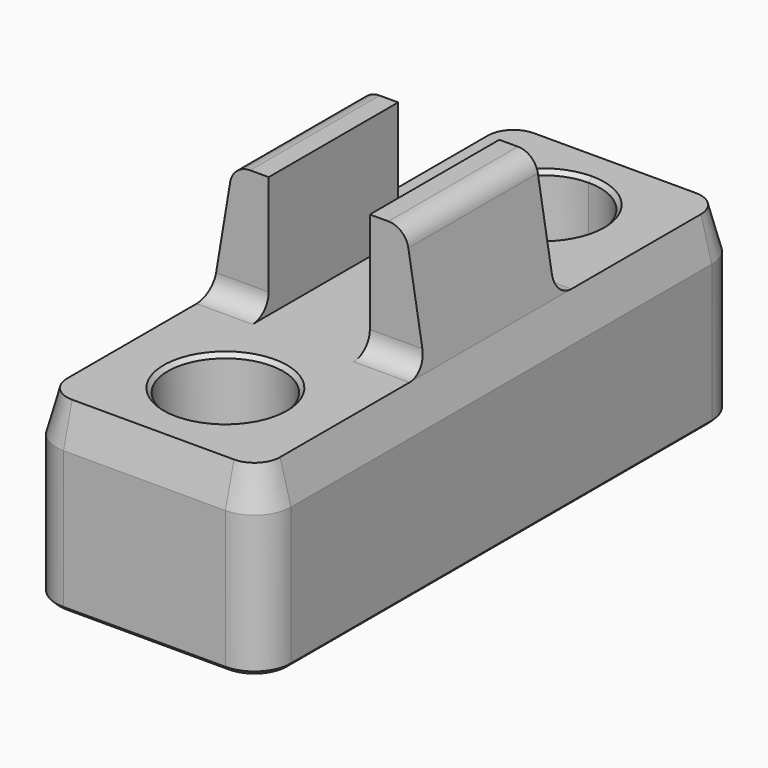
from build123d import *

# Parameters (mm, degrees)
F1_DEPTH      = 9
F3_DEPTH      = 25
F4_DEPTH      = 3.2
F5_SIZE       = 0.2
F6_SIZE2      = 0.5358983849
F6_SIZE       = 2
F7_W          = 2.7641016151
F7_H          = 6
F8_DEPTH      = 6
F9_T4_DEPTH   = 37.1842967295
F9_T9_DEPTH   = 37.1842967295
F10_DEPTH     = 1
F11_DEPTH     = 1
F12_T4_DEPTH  = 5.2641016151
F12_T10_DEPTH = 5.2641016151
F12_T16_DEPTH = 5.2641016151
F12_T22_DEPTH = 5.2641016151
F12_T28_DEPTH = 5.2641016151
F12_T34_DEPTH = 5.2641016151
F12_T40_DEPTH = 5.2641016151
F12_T46_DEPTH = 5.2641016151
F12_T49_DEPTH = 12.2356354419


# Not quite as in the source:
# - a fillet or chamfer that OpenCascade refuses, or shapes differently, is made with other operations: its cross-section is extruded or revolved along the edge and cut away or added


with BuildPart() as f1:
    # F0 (on Top) → F1 (new body)
    with BuildSketch(Plane.XY):
        with BuildLine():
            Line((-34.4771644294, 42.6813552976), (-34.4771644294, 68.6813552976))
            ThreePointArc((-34.4771644294, 68.6813552976), (-35.0043722233, 69.9541475037), (-36.2771644294, 70.4813552976))
            Line((-36.2771644294, 70.4813552976), (-44.2771644294, 70.4813552976))
            ThreePointArc((-44.2771644294, 70.4813552976), (-45.5499566356, 69.9541475037), (-46.0771644294, 68.6813552976))
            Line((-46.0771644294, 68.6813552976), (-46.0771644294, 42.6813552976))
            ThreePointArc((-46.0771644294, 42.6813552976), (-45.5499566356, 41.4085630914), (-44.2771644294, 40.8813552976))
            Line((-44.2771644294, 40.8813552976), (-36.2771644294, 40.8813552976))
            ThreePointArc((-36.2771644294, 40.8813552976), (-35.0043722233, 41.4085630914), (-34.4771644294, 42.6813552976))
        make_face()
    extrude(amount=F1_DEPTH)

    # F2 (on face) → F3 (cut)
    with BuildSketch(Plane.XY.offset(9)):
        with BuildLine():
            ThreePointArc((-38.7771644294, 65.4813552976), (-39.2165042576, 66.5420154693), (-40.2771644294, 66.9813552976))
            ThreePointArc((-40.2771644294, 66.9813552976), (-41.3378246012, 64.4206951258), (-38.7771644294, 65.4813552976))
        make_face()
        with BuildLine():
            ThreePointArc((-38.7771644294, 45.8813552976), (-41.3378246012, 46.9420154693), (-40.2771644294, 44.3813552976))
            ThreePointArc((-40.2771644294, 44.3813552976), (-39.2165042576, 44.8206951258), (-38.7771644294, 45.8813552976))
        make_face()
    extrude(amount=-F3_DEPTH, mode=Mode.SUBTRACT)

    # F2 (on face) → F4 (cut)
    with BuildSketch(Plane.XY.offset(9)):
        with BuildLine():
            ThreePointArc((-37.4271644294, 65.4813552976), (-38.261910103, 67.4966096239), (-40.2771644294, 68.3313552976))
            ThreePointArc((-40.2771644294, 68.3313552976), (-42.2924187558, 63.4661009712), (-37.4271644294, 65.4813552976))
        make_face()
        with BuildLine():
            ThreePointArc((-38.7771644294, 65.4813552976), (-41.3378246012, 64.4206951258), (-40.2771644294, 66.9813552976))
            ThreePointArc((-40.2771644294, 66.9813552976), (-39.2165042576, 66.5420154693), (-38.7771644294, 65.4813552976))
        make_face(mode=Mode.SUBTRACT)
        with BuildLine():
            ThreePointArc((-37.4271644294, 45.8813552976), (-42.2924187558, 47.8966096239), (-40.2771644294, 43.0313552976))
            ThreePointArc((-40.2771644294, 43.0313552976), (-38.261910103, 43.8661009712), (-37.4271644294, 45.8813552976))
        make_face()
        with BuildLine():
            ThreePointArc((-38.7771644294, 45.8813552976), (-39.2165042576, 44.8206951258), (-40.2771644294, 44.3813552976))
            ThreePointArc((-40.2771644294, 44.3813552976), (-41.3378246012, 46.9420154693), (-38.7771644294, 45.8813552976))
        make_face(mode=Mode.SUBTRACT)
    extrude(amount=-F4_DEPTH, mode=Mode.SUBTRACT)

    # F5
    f5_edges = [f1.edges().sort_by_distance(p)[0] for p in [
        (-40.277164, 63.981355, 5.8),
        (-40.277164, 47.381355, 5.8),
        (-34.477164, 55.681355, 0),
        (-35.004372, 41.408563, 0),
        (-35.004372, 69.954148, 0),
        (-40.277164, 40.881355, 0),
        (-40.277164, 70.481355, 0),
        (-45.549957, 41.408563, 0),
        (-45.549957, 69.954148, 0),
        (-46.077164, 55.681355, 0),
        (-40.277164, 47.381355, 0),
        (-40.277164, 63.981355, 0),
        (-40.277164, 62.631355, 9),
        (-40.277164, 48.731355, 9),
    ]]
    chamfer(f5_edges, length=F5_SIZE)

    # F6
    f6_edges = [f1.edges().sort_by_distance(p)[0] for p in [
        (-34.477164, 55.681355, 9),
    ]]
    f6_side = f1.faces().sort_by_distance((-34.477164, 55.681355, 4.6))[0]
    chamfer(f6_edges, length=F6_SIZE, length2=F6_SIZE2, reference=f6_side)

    # F7 (on face) → F8 (join)
    with BuildSketch(Plane.XY.offset(9)):
        with Locations((-36.3951136219, 55.6813552976)):
            Rectangle(F7_W, F7_H)
        with Locations((-44.159215237, 55.6813552976)):
            Rectangle(F7_W, F7_H)
    extrude(amount=F8_DEPTH)

    # F9: chamfer of 1 x 6 on 2 edges, made by hand


with BuildPart() as f9_tool2:
    # F9_s3 → F9_t4 (new body)
    with BuildSketch(Plane.XZ.offset(-37.0892069328)):
        Polygon((-35.0130628143, 9), (-36.0130628143, 15), (-35.0130628143, 15), align=None)
    extrude(amount=-F9_T4_DEPTH)

    split(bisect_by=Plane(origin=(-30.4176323379, 0, -8.1503800206), x_dir=(0, 1, 0), z_dir=(0.9659258263, 0, 0.2588190451)), keep=Keep.TOP)


with BuildPart() as f1_1:
    add(f1.part)

    # F9_t1: cut F9_tool2
    add(f9_tool2.part, mode=Mode.SUBTRACT)


with BuildPart() as f9_tool7:
    # F9_s8 → F9_t9 (new body)
    with BuildSketch(Plane.XZ.offset(-74.2735036623)):
        Polygon((-45.5412660446, 9), (-44.5412660446, 15), (-45.5412660446, 15), align=None)
    extrude(amount=F9_T9_DEPTH)

    split(bisect_by=Plane(origin=(-44.7405796798, 0, 11.9882021941), x_dir=(0, 1, 0), z_dir=(-0.9659258263, 0, 0.2588190451)), keep=Keep.TOP)


with BuildPart() as f1_2:
    add(f1_1.part)

    # F9_t6: cut F9_tool7
    add(f9_tool7.part, mode=Mode.SUBTRACT)

    # F10 (add): faces of the model
    f10_faces = [f1_2.faces().sort_by_distance(p)[0] for p in [
        (-36.6267104431, 58.6813552976, 11.7791618553),
        (-43.9276184157, 58.6813552976, 11.7791618553),
    ]]
    extrude(f10_faces, amount=F10_DEPTH)

    # F11 (add): faces of the model
    f11_faces = [f1_2.faces().sort_by_distance(p)[0] for p in [
        (-43.9276184157, 52.6813552976, 11.7791618553),
        (-36.6267104431, 52.6813552976, 11.7791618553),
    ]]
    extrude(f11_faces, amount=F11_DEPTH)

    # F12: fillet of radius 1 on 6 edges, made by hand


with BuildPart() as f12_tool2:
    # F12_s3 → F12_t4 (new body)
    with BuildSketch(Plane.YZ.offset(-37.7771644294)):
        with BuildLine():
            ThreePointArc((50.6813552976, 9), (51.3884620788, 9.2928932188), (51.6813552976, 10))
            Line((51.6813552976, 10), (51.6813552976, 9))
            Line((51.6813552976, 9), (50.6813552976, 9))
        make_face()
    extrude(amount=F12_T4_DEPTH)

    split(bisect_by=Plane(origin=(-30.4176323379, 0, -8.1503800206), x_dir=(0, 1, 0), z_dir=(-0.9659258263, 0, -0.2588190451)), keep=Keep.TOP)

    split(bisect_by=Plane(origin=(-32.6073043599, 0, -5.4345507266), x_dir=(0, 1, 0), z_dir=(-0.9863939238, 0, -0.1643989873)), keep=Keep.TOP)


with BuildPart() as f1_3:
    add(f1_2.part)

    # F12_t1: union F12_tool2
    add(f12_tool2.part)


with BuildPart() as f12_tool8:
    # F12_s9 → F12_t10 (new body)
    with BuildSketch(Plane.YZ.offset(-37.7771644294)):
        with BuildLine():
            ThreePointArc((50.6813552976, 9), (51.3884620788, 9.2928932188), (51.6813552976, 10))
            Line((51.6813552976, 10), (51.6813552976, 9))
            Line((51.6813552976, 9), (50.6813552976, 9))
        make_face()
    extrude(amount=F12_T10_DEPTH)

    split(bisect_by=Plane(origin=(-30.4176323379, 0, -8.1503800206), x_dir=(0, 1, 0), z_dir=(0.9659258263, 0, 0.2588190451)), keep=Keep.TOP)

    split(bisect_by=Plane(origin=(-32.6073043599, 0, -5.4345507266), x_dir=(0, 1, 0), z_dir=(-0.9863939238, 0, -0.1643989873)), keep=Keep.TOP)


with BuildPart() as f1_4:
    add(f1_3.part)

    # F12_t7: union F12_tool8
    add(f12_tool8.part)


with BuildPart() as f12_tool14:
    # F12_s15 → F12_t16 (new body)
    with BuildSketch(Plane.YZ.offset(-48.0412660446)):
        with BuildLine():
            ThreePointArc((50.6813552976, 9), (51.3884620788, 9.2928932188), (51.6813552976, 10))
            Line((51.6813552976, 10), (51.6813552976, 9))
            Line((51.6813552976, 9), (50.6813552976, 9))
        make_face()
    extrude(amount=F12_T16_DEPTH)

    split(bisect_by=Plane(origin=(-44.7405796798, 0, 11.9882021941), x_dir=(0, 1, 0), z_dir=(-0.9659258263, 0, 0.2588190451)), keep=Keep.TOP)

    split(bisect_by=Plane(origin=(-45.7698804758, 0, 7.6283134126), x_dir=(0, 1, 0), z_dir=(0.9863939238, 0, -0.1643989873)), keep=Keep.TOP)


with BuildPart() as f1_5:
    add(f1_4.part)

    # F12_t13: union F12_tool14
    add(f12_tool14.part)


with BuildPart() as f12_tool20:
    # F12_s21 → F12_t22 (new body)
    with BuildSketch(Plane.YZ.offset(-48.0412660446)):
        with BuildLine():
            ThreePointArc((50.6813552976, 9), (51.3884620788, 9.2928932188), (51.6813552976, 10))
            Line((51.6813552976, 10), (51.6813552976, 9))
            Line((51.6813552976, 9), (50.6813552976, 9))
        make_face()
    extrude(amount=F12_T22_DEPTH)

    split(bisect_by=Plane(origin=(-44.7405796798, 0, 11.9882021941), x_dir=(0, 1, 0), z_dir=(0.9659258263, 0, -0.2588190451)), keep=Keep.TOP)

    split(bisect_by=Plane(origin=(-45.7698804758, 0, 7.6283134126), x_dir=(0, 1, 0), z_dir=(0.9863939238, 0, -0.1643989873)), keep=Keep.TOP)


with BuildPart() as f1_6:
    add(f1_5.part)

    # F12_t19: union F12_tool20
    add(f12_tool20.part)


with BuildPart() as f12_tool26:
    # F12_s27 → F12_t28 (new body)
    with BuildSketch(Plane.YZ.offset(-32.5130628143)):
        with BuildLine():
            ThreePointArc((60.6813552976, 9), (59.9742485164, 9.2928932188), (59.6813552976, 10))
            Line((59.6813552976, 10), (59.6813552976, 9))
            Line((59.6813552976, 9), (60.6813552976, 9))
        make_face()
    extrude(amount=-F12_T28_DEPTH)

    split(bisect_by=Plane(origin=(-30.4176323379, 0, -8.1503800206), x_dir=(0, 1, 0), z_dir=(0.9659258263, 0, 0.2588190451)), keep=Keep.TOP)

    split(bisect_by=Plane(origin=(-32.6073043599, 0, -5.4345507266), x_dir=(0, 1, 0), z_dir=(-0.9863939238, 0, -0.1643989873)), keep=Keep.TOP)


with BuildPart() as f1_7:
    add(f1_6.part)

    # F12_t25: union F12_tool26
    add(f12_tool26.part)


with BuildPart() as f12_tool32:
    # F12_s33 → F12_t34 (new body)
    with BuildSketch(Plane.YZ.offset(-32.5130628143)):
        with BuildLine():
            ThreePointArc((60.6813552976, 9), (59.9742485164, 9.2928932188), (59.6813552976, 10))
            Line((59.6813552976, 10), (59.6813552976, 9))
            Line((59.6813552976, 9), (60.6813552976, 9))
        make_face()
    extrude(amount=-F12_T34_DEPTH)

    split(bisect_by=Plane(origin=(-30.4176323379, 0, -8.1503800206), x_dir=(0, 1, 0), z_dir=(-0.9659258263, 0, -0.2588190451)), keep=Keep.TOP)

    split(bisect_by=Plane(origin=(-32.6073043599, 0, -5.4345507266), x_dir=(0, 1, 0), z_dir=(-0.9863939238, 0, -0.1643989873)), keep=Keep.TOP)


with BuildPart() as f1_8:
    add(f1_7.part)

    # F12_t31: union F12_tool32
    add(f12_tool32.part)


with BuildPart() as f12_tool38:
    # F12_s39 → F12_t40 (new body)
    with BuildSketch(Plane.YZ.offset(-42.7771644294)):
        with BuildLine():
            ThreePointArc((60.6813552976, 9), (59.9742485164, 9.2928932188), (59.6813552976, 10))
            Line((59.6813552976, 10), (59.6813552976, 9))
            Line((59.6813552976, 9), (60.6813552976, 9))
        make_face()
    extrude(amount=-F12_T40_DEPTH)

    split(bisect_by=Plane(origin=(-44.7405796798, 0, 11.9882021941), x_dir=(0, 1, 0), z_dir=(0.9659258263, 0, -0.2588190451)), keep=Keep.TOP)

    split(bisect_by=Plane(origin=(-45.7698804758, 0, 7.6283134126), x_dir=(0, 1, 0), z_dir=(0.9863939238, 0, -0.1643989873)), keep=Keep.TOP)


with BuildPart() as f1_9:
    add(f1_8.part)

    # F12_t37: union F12_tool38
    add(f12_tool38.part)


with BuildPart() as f12_tool44:
    # F12_s45 → F12_t46 (new body)
    with BuildSketch(Plane.YZ.offset(-42.7771644294)):
        with BuildLine():
            ThreePointArc((60.6813552976, 9), (59.9742485164, 9.2928932188), (59.6813552976, 10))
            Line((59.6813552976, 10), (59.6813552976, 9))
            Line((59.6813552976, 9), (60.6813552976, 9))
        make_face()
    extrude(amount=-F12_T46_DEPTH)

    split(bisect_by=Plane(origin=(-44.7405796798, 0, 11.9882021941), x_dir=(0, 1, 0), z_dir=(-0.9659258263, 0, 0.2588190451)), keep=Keep.TOP)

    split(bisect_by=Plane(origin=(-45.7698804758, 0, 7.6283134126), x_dir=(0, 1, 0), z_dir=(0.9863939238, 0, -0.1643989873)), keep=Keep.TOP)


with BuildPart() as f1_10:
    add(f1_9.part)

    # F12_t43: union F12_tool44
    add(f12_tool44.part)

    # F12_s50 → F12_t49 (cut)
    with BuildSketch(Plane.XZ.offset(-61.7991730185)):
        with BuildLine():
            ThreePointArc((-36.8601899027, 15), (-36.2138150066, 14.7630199825), (-35.8737959789, 14.1643989873))
            Line((-35.8737959789, 14.1643989873), (-36.0130628143, 15))
            Line((-36.0130628143, 15), (-36.8601899027, 15))
        make_face()
        with BuildLine():
            ThreePointArc((-44.68053288, 14.1643989873), (-44.3405138523, 14.7630199825), (-43.6941389562, 15))
            Line((-43.6941389562, 15), (-44.5412660446, 15))
            Line((-44.5412660446, 15), (-44.68053288, 14.1643989873))
        make_face()
    extrude(amount=F12_T49_DEPTH, mode=Mode.SUBTRACT)


solid = f1_10.part
